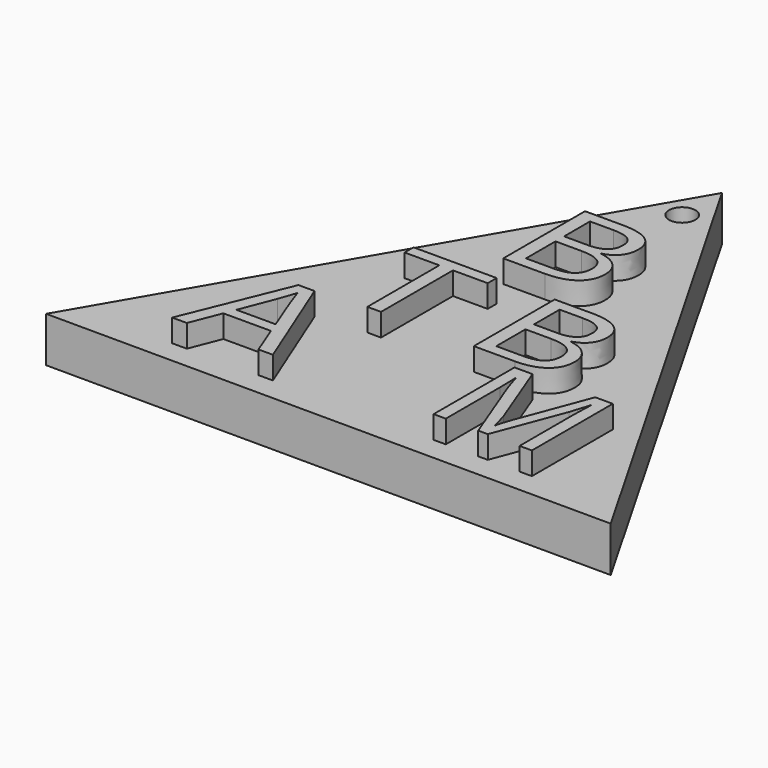
from build123d import *

# Parameters (mm, degrees)
F0_R           = 1.1626869356
F2_DEPTH       = 4
F1_TEXT_SIZE   = 13.1207996876
F1_TEXT_SIZE_2 = 12.9826851965
F1_TEXT_SIZE_3 = 13.4218464761
F3_DEPTH       = 6


# Not quite as in the source:
# - Text() gives the source's letters only with a copy of the font that has no kerning and outlines rounded to 1/6400 em; it was checked with that copy


with BuildPart() as f2:
    # F0 (on Top) → F2 (new body)
    with BuildSketch(Plane.XY):
        Polygon((0.0842891032, 22.7222488499), (-25.0420379816, -20.50584025), (24.9577488784, -20.6518332593), align=None)
        with Locations((0, 18.4354246594)):
            Circle(F0_R, mode=Mode.SUBTRACT)
    extrude(amount=F2_DEPTH)

    # F1 (on Top) → F3 (join)
    with BuildSketch(Plane.XY):
        with Locations((-4.2631055694, 2.6648738421)):
            Text('B', F1_TEXT_SIZE, font='Arimo', text_align=(TextAlign.LEFT, TextAlign.BOTTOM))
        with Locations((-9.343446116, -8.845763281)):
            Text('T', F1_TEXT_SIZE_2, font='Arimo', text_align=(TextAlign.LEFT, TextAlign.BOTTOM))
        with Locations((2.3534579668, -8.845763281)):
            Text('B', F1_TEXT_SIZE_2, font='Arimo', text_align=(TextAlign.LEFT, TextAlign.BOTTOM))
        with Locations((-15.5260779296, -18.5094927438)):
            Text('A', F1_TEXT_SIZE_3, font='Arimo', text_align=(TextAlign.LEFT, TextAlign.BOTTOM))
        with Locations((6.5328529937, -18.5094927438)):
            Text('M', F1_TEXT_SIZE_2, font='Arimo', text_align=(TextAlign.LEFT, TextAlign.BOTTOM))
    extrude(amount=F3_DEPTH)


solid = f2.part
